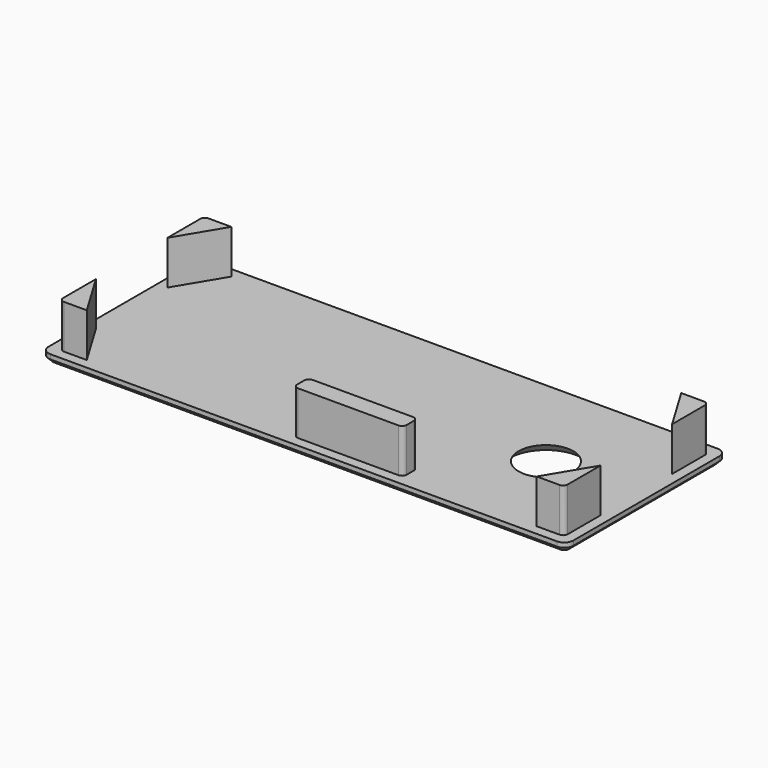
from build123d import *

# Parameters (mm, degrees)
F0_R     = 3
F1_DEPTH = 1
F3_DEPTH = 4.8
F4_SIZE  = 0.99999
F5_SIZE  = 0.5


# Not quite as in the source:
# - a fillet or chamfer is up to 0.001 mm smaller than in the source, because OpenCascade refuses the exact size


with BuildPart() as f1:
    # F0 (on Top) → F1 (new body)
    with BuildSketch(Plane.XY):
        with BuildLine():
            Line((56.5, 22), (1, 22))
            ThreePointArc((1, 22), (0.2928932188, 21.7071067812), (0, 21))
            Line((0, 21), (0, 1))
            ThreePointArc((0, 1), (0.2928932188, 0.2928932188), (1, 0))
            Line((1, 0), (56.5, 0))
            ThreePointArc((56.5, 0), (57.2071067812, 0.2928932188), (57.5, 1))
            Line((57.5, 1), (57.5, 21))
            ThreePointArc((57.5, 21), (57.2071067812, 21.7071067812), (56.5, 22))
        make_face()
        with Locations((46.5, 11)):
            Circle(F0_R, mode=Mode.SUBTRACT)
    extrude(amount=F1_DEPTH)

    # F2 (on face) → F3 (join)
    with BuildSketch(Plane.XY.offset(1)):
        with BuildLine():
            Line((1.1, 20.4), (1.1, 15.9))
            Line((1.1, 15.9), (4.1, 20.9))
            Line((4.1, 20.9), (1.6, 20.9))
            ThreePointArc((1.6, 20.9), (1.2464466094, 20.7535533906), (1.1, 20.4))
        make_face()
        with BuildLine():
            ThreePointArc((56.4, 20.4), (56.2535533906, 20.7535533906), (55.9, 20.9))
            Line((55.9, 20.9), (53.4, 20.9))
            Line((53.4, 20.9), (56.4, 15.9))
            Line((56.4, 15.9), (56.4, 20.4))
        make_face()
        with BuildLine():
            ThreePointArc((1.1, 1.6), (1.2464466094, 1.2464466094), (1.6, 1.1))
            Line((1.6, 1.1), (4.1, 1.1))
            Line((4.1, 1.1), (1.1, 6.1))
            Line((1.1, 6.1), (1.1, 1.6))
        make_face()
        with BuildLine():
            Line((53.4, 1.1), (55.9, 1.1))
            ThreePointArc((55.9, 1.1), (56.2535533906, 1.2464466094), (56.4, 1.6))
            Line((56.4, 1.6), (56.4, 6.1))
            Line((56.4, 6.1), (53.4, 1.1))
        make_face()
        with BuildLine():
            Line((38.25, 3.1), (27.25, 3.1))
            ThreePointArc((27.25, 3.1), (26.8964466094, 2.9535533906), (26.75, 2.6))
            Line((26.75, 2.6), (26.75, 1.6))
            ThreePointArc((26.75, 1.6), (26.8964466094, 1.2464466094), (27.25, 1.1))
            Line((27.25, 1.1), (38.25, 1.1))
            ThreePointArc((38.25, 1.1), (38.6035533906, 1.2464466094), (38.75, 1.6))
            Line((38.75, 1.6), (38.75, 2.6))
            ThreePointArc((38.75, 2.6), (38.6035533906, 2.9535533906), (38.25, 3.1))
        make_face()
    extrude(amount=F3_DEPTH)

    # F4 (size 1 in the source; OpenCascade refuses exactly that, so slightly less here)
    f4_edges = [f1.edges().sort_by_distance(p)[0] for p in [
        (43.5, 11, 0),
    ]]
    chamfer(f4_edges, length=F4_SIZE)

    # F5
    f5_edges = [f1.edges().sort_by_distance(p)[0] for p in [
        (28.75, 0, 0),
        (0, 11, 0),
        (0.292893, 0.292893, 0),
        (0.292893, 21.707107, 0),
        (28.75, 22, 0),
        (57.5, 11, 0),
        (57.207107, 0.292893, 0),
        (57.207107, 21.707107, 0),
    ]]
    chamfer(f5_edges, length=F5_SIZE)


solid = f1.part
